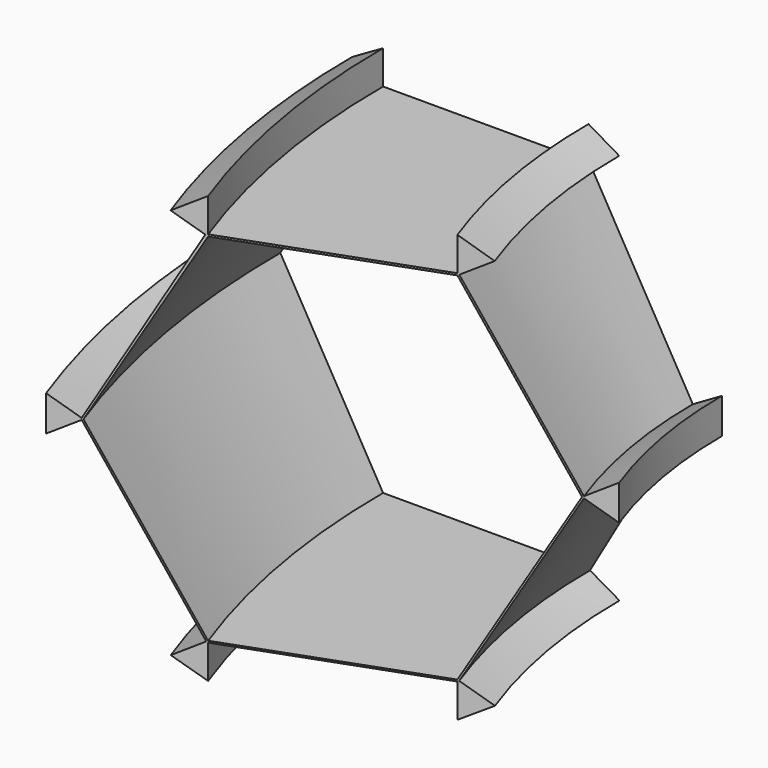
from build123d import *

# Parameters (mm, degrees)
F1_W     = 14.6656349089
F1_H     = 0.1217532289
F2_ANGLE = 20


with BuildPart() as f2:
    # F1 (on Front) → F2 (revolve)
    with BuildSketch(Plane.XZ):
        Polygon((-43.7767438772, 12.7751471548), (-43.8843175875, 12.7008123937), (-43.7714494091, 12.7659768669), align=None)
        Polygon((-36.4386319546, 0.0651644732), (-36.5515001331, 0), (-36.4439264228, -0.0621077106), (-36.3309057177, -0.1273602451), (-34.3620503103, -1.2640794445), (-34.3620503103, 1.2640794445), align=None)
        Polygon((-58.7149140006, 12.7960529626), (-58.5499524964, 12.7008123937), (-58.5499524964, 12.8391478211), (-58.5499524964, 15.2491778135), (-60.7598529608, 13.9766990217), align=None)
        Polygon((-43.7767438772, -12.7629201043), (-43.8843175875, -12.7008123937), (-43.8843175875, -12.8225656226), (-43.8843175875, -15.2283469215), (-41.6742515512, -13.9767946147), align=None)
        Polygon((-58.5499524964, -12.8225656226), (-58.5499524964, -12.7008123937), (-58.6575262067, -12.7629201043), (-60.7503676631, -13.9712226825), (-58.5499524964, -15.2283469215), align=None)
        Polygon((-65.9903436611, -0.0621077106), (-65.8827699508, 0), (-65.9900653034, 0.0619470007), (-68.0832503253, 1.2704479365), (-68.0832503253, -1.2704479365), align=None)
        Polygon((-43.8843175875, 12.7008123937), (-36.5515001331, 0), (-36.4386319546, 0.0651644732), (-43.7714494091, 12.7659768669), align=None)
        Polygon((-36.5515001331, 0), (-43.8843175875, -12.7008123937), (-43.7767438772, -12.7629201043), (-36.4439264228, -0.0621077106), align=None)
        Polygon((-58.5499524964, 12.8391478211), (-58.5499524964, 12.7008123937), (-51.217135042, 12.7008123937), (-43.8843175875, 12.7008123937), (-43.8843175875, 12.8391478211), align=None)
        Polygon((-43.8843175875, 15.2525296435), (-43.8843175875, 12.8391478211), (-43.8843175875, 12.7008123937), (-43.7767438772, 12.7751471548), (-43.7714494091, 12.7659768669), (-41.6910577545, 13.9670915487), align=None)
        Polygon((-65.9900653034, 0.0619470007), (-65.8827699508, 0), (-58.5499524964, 12.7008123937), (-58.7149140006, 12.7960529626), align=None)
        with Locations((-51.217135042, -12.7616890082)):
            Rectangle(F1_W, F1_H)
        Polygon((-58.5499524964, -12.7008123937), (-65.8827699508, 0), (-65.9903436611, -0.0621077106), (-65.9526700928, -0.1273602451), (-58.6575262067, -12.7629201043), align=None)
    revolve(axis=Axis((0, 0, 0), (0, 0, 1)), revolution_arc=F2_ANGLE)


solid = f2.part
